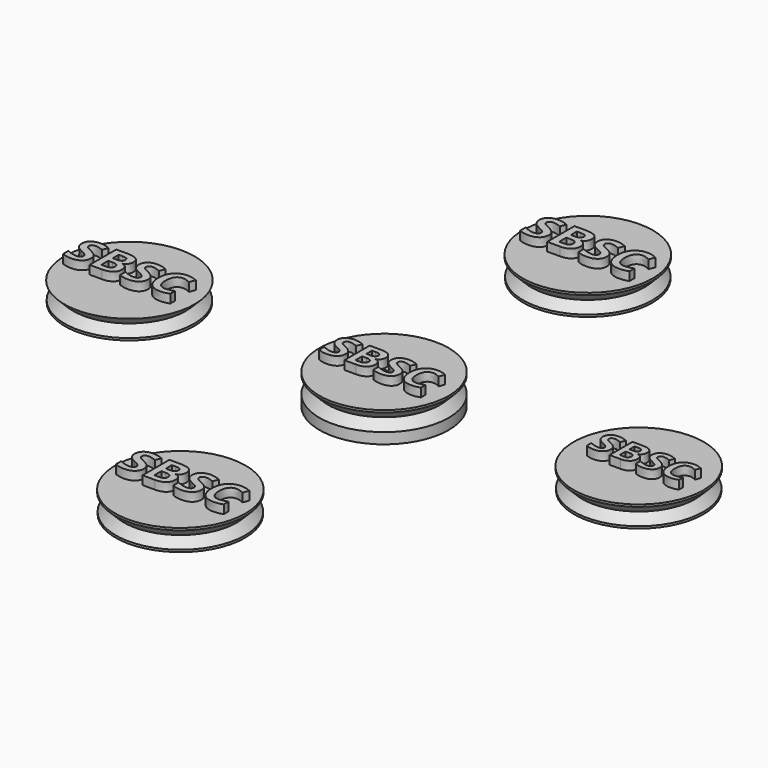
from build123d import *

# Parameters (mm, degrees)
F0_R            = 15
F1_DEPTH        = 2.5
F3_SIZE         = 2
F3_2_SIZE       = 2
F3_3_SIZE       = 2
F3_4_SIZE       = 2
F3_5_SIZE       = 2
F2_R            = 15
F2_R_2          = 0.75
F4_DEPTH        = 2.5
F5_SIZE         = 1.99999
F6_R            = 15.1
F6_R_2          = 13
F7_DEPTH        = 2.5
F8_SIZE         = 2
F9_R            = 15.1
F9_R_2          = 13
F10_DEPTH       = 2
F11_SIZE        = 1.99999
F12_R           = 15.1
F13_DEPTH       = 2.5
F14_SIZE        = 2
F15_R           = 15.1
F16_DEPTH       = 2.5
F17_SIZE        = 2
F19_TEXT_SIZE   = 9.3040370201
F19_TEXT_SIZE_2 = 10.8963809907
F19_TEXT_SIZE_3 = 10.8304805407
F19_TEXT_SIZE_4 = 11.0485435774
F18_TEXT_SIZE   = 10.2796055014
F20_DEPTH       = 2
F21_DEPTH       = 2


# Not quite as in the source:
# - a fillet or chamfer is up to 0.001 mm smaller than in the source, because OpenCascade refuses the exact size
# - Text() gives the source's letters only with a copy of the font that has no kerning and outlines rounded to 1/6400 em; it was checked with that copy


with BuildPart() as f1:
    # F0 (on Top) → F1 (new body)
    with BuildSketch(Plane.XY):
        Circle(F0_R)
    extrude(amount=F1_DEPTH)

    # F3
    f3_edges = [f1.edges().sort_by_distance(p)[0] for p in [
        (-15, 0, 2.5),
    ]]
    chamfer(f3_edges, length=F3_SIZE)

    # F2 (on face) → F4 (join)
    with BuildSketch(Plane.XY.offset(2.5)):
        Circle(F2_R)
        Circle(F2_R_2, mode=Mode.SUBTRACT)
    extrude(amount=F4_DEPTH)

    # F5 (size 2 in the source; OpenCascade refuses exactly that, so slightly less here)
    f5_edges = [f1.edges().sort_by_distance(p)[0] for p in [
        (-15, 0, 2.5),
    ]]
    chamfer(f5_edges, length=F5_SIZE)

    # F0 (on Top) → F21 (join)
    with BuildSketch(Plane.XY):
        Circle(F0_R)
    extrude(amount=-F21_DEPTH)


with BuildPart() as f1b:
    # F0 (on Top) → F1, piece 2 (new body)
    with BuildSketch(Plane.XY):
        with Locations((-59.0641727244, 0)):
            Circle(F0_R)
    extrude(amount=F1_DEPTH)

    # F3#4
    f3_4_edges = [f1b.edges().sort_by_distance(p)[0] for p in [
        (-74.064173, 0, 2.5),
    ]]
    chamfer(f3_4_edges, length=F3_4_SIZE)

    # F9 (on face) → F10 (join)
    with BuildSketch(Plane.XY.offset(2.5)):
        with Locations((-59.0641727244, 0)):
            Circle(F9_R)
        with Locations((-59.0641727244, 0)):
            Circle(F9_R_2, mode=Mode.SUBTRACT)
        with Locations((-59.0641727244, 0)):
            Circle(F9_R_2)
    extrude(amount=F10_DEPTH)

    # F11 (size 2 in the source; OpenCascade refuses exactly that, so slightly less here)
    f11_edges = [f1b.edges().sort_by_distance(p)[0] for p in [
        (-74.164173, 0, 2.5),
    ]]
    chamfer(f11_edges, length=F11_SIZE)


with BuildPart() as f1c:
    # F0 (on Top) → F1, piece 3 (new body)
    with BuildSketch(Plane.XY):
        with Locations((0, 59.0641727244)):
            Circle(F0_R)
    extrude(amount=F1_DEPTH)

    # F3#5
    f3_5_edges = [f1c.edges().sort_by_distance(p)[0] for p in [
        (-15, 59.064173, 2.5),
    ]]
    chamfer(f3_5_edges, length=F3_5_SIZE)

    # F6 (on face) → F7 (join)
    with BuildSketch(Plane.XY.offset(2.5)):
        with Locations((0, 59.0641727244)):
            Circle(F6_R)
        with Locations((0, 59.0641727244)):
            Circle(F6_R_2, mode=Mode.SUBTRACT)
        with Locations((0, 59.0641727244)):
            Circle(F6_R_2)
    extrude(amount=F7_DEPTH)

    # F8
    f8_edges = [f1c.edges().sort_by_distance(p)[0] for p in [
        (-15.1, 59.064173, 2.5),
    ]]
    chamfer(f8_edges, length=F8_SIZE)


with BuildPart() as f1d:
    # F0 (on Top) → F1, piece 4 (new body)
    with BuildSketch(Plane.XY):
        with Locations((0, -59.0641727244)):
            Circle(F0_R)
    extrude(amount=F1_DEPTH)

    # F3#3
    f3_3_edges = [f1d.edges().sort_by_distance(p)[0] for p in [
        (-15, -59.064173, 2.5),
    ]]
    chamfer(f3_3_edges, length=F3_3_SIZE)

    # F12 (on face) → F13 (join)
    with BuildSketch(Plane.XY.offset(2.5)):
        with Locations((0, -59.0641727244)):
            Circle(F12_R)
    extrude(amount=F13_DEPTH)

    # F14
    f14_edges = [f1d.edges().sort_by_distance(p)[0] for p in [
        (-15.1, -59.064173, 2.5),
    ]]
    chamfer(f14_edges, length=F14_SIZE)


with BuildPart() as f1e:
    # F0 (on Top) → F1, piece 5 (new body)
    with BuildSketch(Plane.XY):
        with Locations((59.0641727244, 0)):
            Circle(F0_R)
    extrude(amount=F1_DEPTH)

    # F3#2
    f3_2_edges = [f1e.edges().sort_by_distance(p)[0] for p in [
        (44.064173, 0, 2.5),
    ]]
    chamfer(f3_2_edges, length=F3_2_SIZE)

    # F15 (on face) → F16 (join)
    with BuildSketch(Plane.XY.offset(2.5)):
        with Locations((59.0641727244, 0)):
            Circle(F15_R)
    extrude(amount=F16_DEPTH)

    # F17
    f17_edges = [f1e.edges().sort_by_distance(p)[0] for p in [
        (43.964173, 0, 2.5),
    ]]
    chamfer(f17_edges, length=F17_SIZE)


with BuildPart() as f20:
    # F19 (on face) + F18 (on face) → F20 (new body)
    with BuildSketch(Plane.XY.offset(5)):
        with Locations((48.7167090178, -2.9548108578)):
            Text('SBSC', F19_TEXT_SIZE, font='Open Sans', font_style=FontStyle.BOLD, text_align=(TextAlign.LEFT, TextAlign.BOTTOM))
        with Locations((-13.4034302027, -62.004558742)):
            Text('SBSC', F19_TEXT_SIZE_2, font='Open Sans', font_style=FontStyle.BOLD, text_align=(TextAlign.LEFT, TextAlign.BOTTOM))
        with Locations((-72.4119916558, -3.5390523262)):
            Text('SBSC', F19_TEXT_SIZE_3, font='Open Sans', font_style=FontStyle.BOLD, text_align=(TextAlign.LEFT, TextAlign.BOTTOM))
        with Locations((-13.4809494994, 55.3100556135)):
            Text('SBSC', F19_TEXT_SIZE_4, font='Open Sans', font_style=FontStyle.BOLD, text_align=(TextAlign.LEFT, TextAlign.BOTTOM))
    with BuildSketch(Plane.XY.offset(5)):
        with Locations((-12.6645918936, -3.9099988062)):
            Text('SBSC', F18_TEXT_SIZE, font='Open Sans', font_style=FontStyle.BOLD, text_align=(TextAlign.LEFT, TextAlign.BOTTOM))
    extrude(amount=F20_DEPTH)


solid = Compound([f1.part, f1b.part, f1c.part, f1d.part, f1e.part, f20.part])
